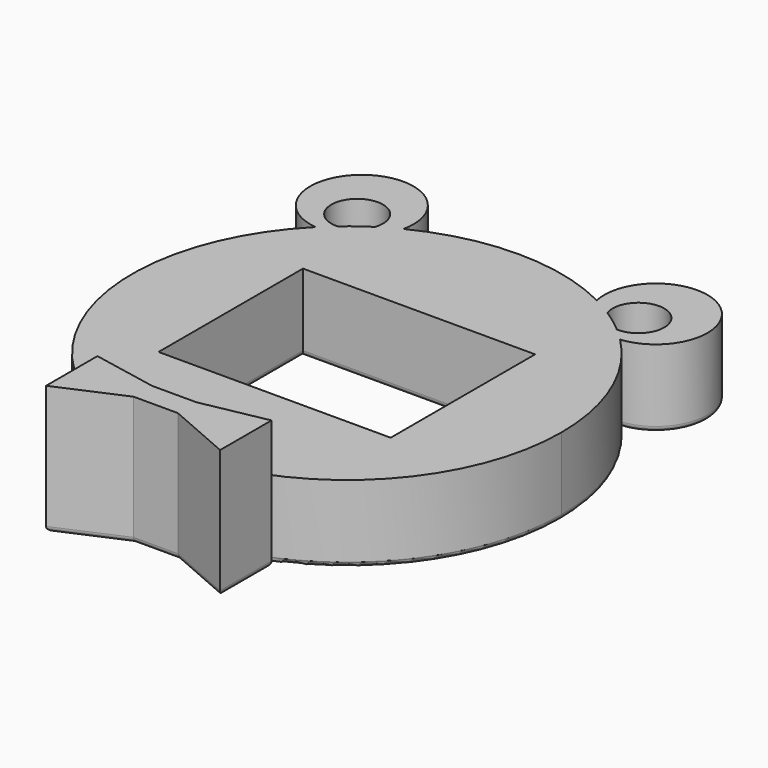
from build123d import *

# Parameters (mm, degrees)
F0_W     = 45
F0_H     = 35
F1_DEPTH = 15
F2_W     = 4.2883176357
F2_H     = 4.5193734479
F3_DEPTH = 25
F4_R     = 5
F5_DEPTH = 2
F6_R     = 1.99999
F6_2_R   = 1.99999
F7_R     = 1
F8_R     = 1


# Not quite as in the source:
# - a fillet or chamfer is up to 0.001 mm smaller than in the source, because OpenCascade refuses the exact size


with BuildPart() as f1:
    # F0 (on Top) → F1 (new body)
    with BuildSketch(Plane.XY):
        with BuildLine():
            ThreePointArc((-29.5201374917, 29.3154231969), (-15.8539921459, -38.4640544896), (41.6032757694, 0))
            ThreePointArc((41.6032757694, 0), (38.4640544896, 15.8539921459), (29.5201374917, 29.3154231969))
            ThreePointArc((29.5201374917, 29.3154231969), (28.3248477073, 30.4718814172), (27.0842908419, 31.5796412952))
            ThreePointArc((27.0842908419, 31.5796412952), (24.8597708938, 33.3590219558), (22.518700562, 34.9820050846))
            ThreePointArc((22.518700562, 34.9820050846), (20.6524683181, 36.1152060372), (18.7293561418, 37.1489404056))
            ThreePointArc((18.7293561418, 37.1489404056), (0, 41.6032757694), (-18.7293561418, 37.1489404056))
            ThreePointArc((-18.7293561418, 37.1489404056), (-20.6524683181, 36.1152060372), (-22.518700562, 34.9820050846))
            ThreePointArc((-22.518700562, 34.9820050846), (-24.8597708938, 33.3590219558), (-27.0842908419, 31.5796412952))
            ThreePointArc((-27.0842908419, 31.5796412952), (-28.3248477073, 30.4718814172), (-29.5201374917, 29.3154231969))
        make_face()
        Rectangle(F0_W, F0_H, mode=Mode.SUBTRACT)
        with BuildLine():
            ThreePointArc((27.0842908419, 31.5796412952), (28.3248477073, 30.4718814172), (29.5201374917, 29.3154231969))
            ThreePointArc((29.5201374917, 29.3154231969), (34.3779025449, 47.3560496198), (18.7293561418, 37.1489404056))
            ThreePointArc((18.7293561418, 37.1489404056), (20.6524683181, 36.1152060372), (22.518700562, 34.9820050846))
            ThreePointArc((22.518700562, 34.9820050846), (30.245316029, 40.5858189836), (27.0842908419, 31.5796412952))
        make_face()
        with BuildLine():
            ThreePointArc((-18.7293561418, 37.1489404056), (-34.3779025449, 47.3560496198), (-29.5201374917, 29.3154231969))
            ThreePointArc((-29.5201374917, 29.3154231969), (-28.3248477073, 30.4718814172), (-27.0842908419, 31.5796412952))
            ThreePointArc((-27.0842908419, 31.5796412952), (-30.245316029, 40.5858189836), (-22.518700562, 34.9820050846))
            ThreePointArc((-22.518700562, 34.9820050846), (-20.6524683181, 36.1152060372), (-18.7293561418, 37.1489404056))
        make_face()
    extrude(amount=F1_DEPTH)

    # F7
    f7_edges = [f1.edges().sort_by_distance(p)[0] for p in [
        (0, -41.603276, 0),
        (-34.377903, 47.35605, 0),
        (0, 41.603276, 0),
        (34.377903, 47.35605, 0),
        (30.245316, 40.585819, 0),
        (24.859771, 33.359022, 0),
        (-30.245316, 40.585819, 0),
        (-24.859771, 33.359022, 0),
        (0, -17.5, 0),
        (22.5, 0, 0),
        (0, 17.5, 0),
        (-22.5, 0, 0),
    ]]
    fillet(f7_edges, radius=F7_R)


with BuildPart() as f3:
    # F2 (on Top) → F3 (new body)
    with BuildSketch(Plane.XY):
        with Locations((2.1441588178, -44.0558715308)):
            Rectangle(F2_W, F2_H)
        with Locations((-2.1441588178, -44.0558715308)):
            Rectangle(F2_W, F2_H)
        Polygon((16.8698690832, -39.3409989774), (4.2883176357, -41.7961848068), (4.2883176357, -46.3155582547), (16.8698690832, -51.7857931554), align=None)
        Polygon((-4.2883176357, -46.3155582547), (-4.2883176357, -41.7961848068), (-16.8698690832, -39.3409989774), (-16.8698690832, -51.7857931554), align=None)
    extrude(amount=F3_DEPTH)

    # F8
    f8_edges = [f3.edges().sort_by_distance(p)[0] for p in [
        (0, -41.796185, 0),
        (-10.579093, -40.568592, 0),
        (-16.869869, -45.563396, 0),
        (-10.579093, -49.050676, 0),
        (0, -46.315558, 0),
        (10.579093, -49.050676, 0),
        (16.869869, -45.563396, 0),
        (10.579093, -40.568592, 0),
    ]]
    fillet(f8_edges, radius=F8_R)


with BuildPart() as f5:
    # F4 (on face) → F5 (new body)
    with BuildSketch(Plane(origin=(0, 0, 0), x_dir=(1, 0, 0), z_dir=(0, 0, -1))):
        with Locations((-10, -30)):
            Circle(F4_R)
    extrude(amount=F5_DEPTH)

    # F6 (radius 2 in the source; OpenCascade refuses exactly that, so slightly less here)
    f6_edges = [f5.edges().sort_by_distance(p)[0] for p in [
        (-15, 30, -2),
    ]]
    fillet(f6_edges, radius=F6_R)


with BuildPart() as f5b:
    # F4 (on face) → F5, piece 2 (new body)
    with BuildSketch(Plane(origin=(0, 0, 0), x_dir=(1, 0, 0), z_dir=(0, 0, -1))):
        with Locations((10, -30)):
            Circle(F4_R)
    extrude(amount=F5_DEPTH)

    # F6#2 (radius 2 in the source; OpenCascade refuses exactly that, so slightly less here)
    f6_2_edges = [f5b.edges().sort_by_distance(p)[0] for p in [
        (5, 30, -2),
    ]]
    fillet(f6_2_edges, radius=F6_2_R)


solid = Compound([f1.part, f3.part, f5.part, f5b.part])
